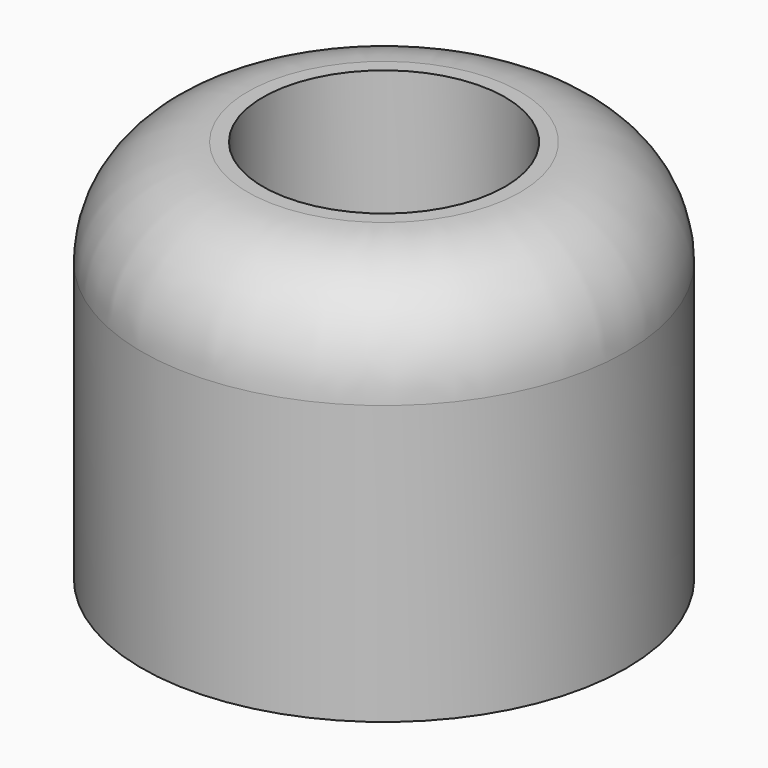
from build123d import *

# Parameters (mm, degrees)
F0_R     = 8
F1_DEPTH = 12.7
F2_R     = 4
F3_DEPTH = 5
F4_D     = 3.2639
F5_R     = 3.5


# Not quite as in the source:
# - a feature names something its author has since deleted; it is built from what else it names


with BuildPart() as f1:
    # F0 (on Top) → F1 (new body)
    with BuildSketch(Plane.XY):
        Circle(F0_R)
    extrude(amount=F1_DEPTH)

    # F2 (on face) → F3 (cut)
    with BuildSketch(Plane.XY.offset(12.7)):
        Circle(F2_R)
    extrude(amount=-F3_DEPTH, mode=Mode.SUBTRACT)

    # F4 (through all)
    with Locations(Plane(origin=(0, 0, 0), x_dir=(1, 0, 0), z_dir=(0, 0, -1))):
        with Locations((0, 0)):
            Hole(F4_D / 2)

    # F5
    f5_edges = [f1.edges().sort_by_distance(p)[0] for p in [
        (-8, 0, 12.7),
    ]]
    fillet(f5_edges, radius=F5_R)


solid = f1.part
